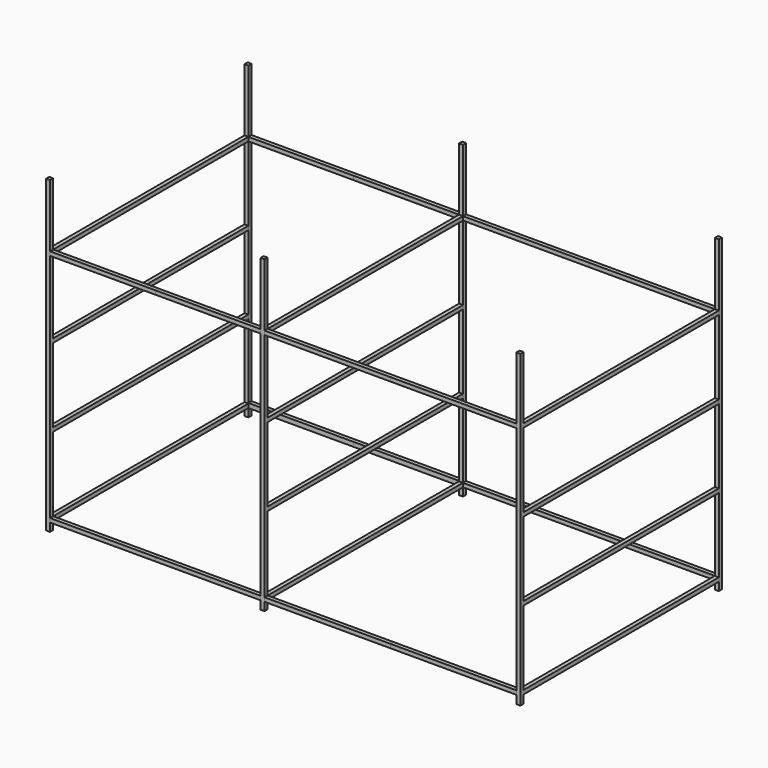
from build123d import *

# Parameters (mm, degrees)
F0_W      = 38.1
F0_H      = 3000
F1_DEPTH  = 38.1
F2_W      = 38.1
F2_H      = 38.1
F3_DEPTH  = 2363.8
F4_W      = 38.1
F4_H      = 38.1
F5_DEPTH  = 2363.8
F6_W      = 38.1
F6_H      = 38.1
F7_DEPTH  = 2363.8
F8_W      = 38.1
F8_H      = 38.1
F9_DEPTH  = 1020
F8_H_2    = 42.8596847504
F11_W     = 38.1
F11_H     = 38.1
F12_DEPTH = 1220


with BuildPart() as f1:
    # F0 (on Right) → F1 (new body)
    with BuildSketch(Plane.YZ):
        with Locations((-185.9003488964, 11.6033870727)):
            Rectangle(F0_W, F0_H)
    extrude(amount=F1_DEPTH)

    # F2 (on face) → F3 (join)
    with BuildSketch(Plane(origin=(0, -166.8503488964, 0), x_dir=(-1, 0, 0), z_dir=(0, 1, 0))):
        with Locations((-19.05, -1389.3466129273)):
            Rectangle(F2_W, F2_H)
    extrude(amount=F3_DEPTH)

    # F4 (on face) → F5 (join)
    with BuildSketch(Plane(origin=(0, -166.8503488964, 0), x_dir=(-1, 0, 0), z_dir=(0, 1, 0))):
        with Locations((-19.05, -631.2466129273)):
            Rectangle(F4_W, F4_H)
    extrude(amount=F5_DEPTH)

    # F6 (on face) → F7 (join)
    with BuildSketch(Plane(origin=(0, -166.8503488964, 0), x_dir=(-1, 0, 0), z_dir=(0, 1, 0))):
        with Locations((-19.05, 126.8533870727)):
            Rectangle(F6_W, F6_H)
        with Locations((-19.05, 884.9533870727)):
            Rectangle(F6_W, F6_H)
    extrude(amount=F7_DEPTH)


with BuildPart() as f1b:
    # F0 (on Right) → F1, piece 2 (new body)
    with BuildSketch(Plane.YZ):
        with Locations((2215.9996511036, 11.6033870727)):
            Rectangle(F0_W, F0_H)
    extrude(amount=F1_DEPTH)


with BuildPart() as f9:
    # F8 (on face) → F9 (new body)
    with BuildSketch(Plane(origin=(0, 0, 0), x_dir=(0, -1, 0), z_dir=(-1, 0, 0))):
        with Locations((185.9003488964, 884.9533870727)):
            Rectangle(F8_W, F8_H)
    extrude(amount=F9_DEPTH)


with BuildPart() as f9b:
    # F8 (on face) → F9, piece 2 (new body)
    with BuildSketch(Plane(origin=(0, 0, 0), x_dir=(0, -1, 0), z_dir=(-1, 0, 0))):
        with Locations((-2215.9996511036, 884.9533870727)):
            Rectangle(F8_W, F8_H)
    extrude(amount=F9_DEPTH)


with BuildPart() as f9c:
    # F8 (on face) → F9, piece 3 (new body)
    with BuildSketch(Plane(origin=(0, 0, 0), x_dir=(0, -1, 0), z_dir=(-1, 0, 0))):
        with Locations((-2215.9996511036, -1386.9667705521)):
            Rectangle(F8_W, F8_H_2)
    extrude(amount=F9_DEPTH)


with BuildPart() as f9d:
    # F8 (on face) → F9, piece 4 (new body)
    with BuildSketch(Plane(origin=(0, 0, 0), x_dir=(0, -1, 0), z_dir=(-1, 0, 0))):
        with Locations((185.9003488964, -1389.3466129273)):
            Rectangle(F8_W, F8_H)
    extrude(amount=F9_DEPTH)


with BuildPart() as f10_1:
    # F10: instance of F1
    add(f1.part.mirror(Plane(origin=(-1020, 2215.9996511036, 884.9533870727), x_dir=(0, -1, 0), z_dir=(-1, 0, 0))))


with BuildPart() as f10_2:
    # F10: instance of F1b
    add(f1b.part.mirror(Plane(origin=(-1020, 2215.9996511036, 884.9533870727), x_dir=(0, -1, 0), z_dir=(-1, 0, 0))))


with BuildPart() as f10_3:
    # F10: instance of F9
    add(f9.part.mirror(Plane(origin=(-1020, 2215.9996511036, 884.9533870727), x_dir=(0, -1, 0), z_dir=(-1, 0, 0))))


with BuildPart() as f10_4:
    # F10: instance of F9b
    add(f9b.part.mirror(Plane(origin=(-1020, 2215.9996511036, 884.9533870727), x_dir=(0, -1, 0), z_dir=(-1, 0, 0))))


with BuildPart() as f10_5:
    # F10: instance of F9c
    add(f9c.part.mirror(Plane(origin=(-1020, 2215.9996511036, 884.9533870727), x_dir=(0, -1, 0), z_dir=(-1, 0, 0))))


with BuildPart() as f10_6:
    # F10: instance of F9d
    add(f9d.part.mirror(Plane(origin=(-1020, 2215.9996511036, 884.9533870727), x_dir=(0, -1, 0), z_dir=(-1, 0, 0))))


with BuildPart() as f12:
    # F11 (on face) → F12 (new body)
    with BuildSketch(Plane.YZ.offset(38.1)):
        with Locations((-185.9003488964, 884.9533870727)):
            Rectangle(F11_W, F11_H)
    extrude(amount=F12_DEPTH)


with BuildPart() as f12b:
    # F11 (on face) → F12, piece 2 (new body)
    with BuildSketch(Plane.YZ.offset(38.1)):
        with Locations((2215.9996511036, 884.9533870727)):
            Rectangle(F11_W, F11_H)
    extrude(amount=F12_DEPTH)


with BuildPart() as f12c:
    # F11 (on face) → F12, piece 3 (new body)
    with BuildSketch(Plane.YZ.offset(38.1)):
        with Locations((-185.9003488964, -1389.3466129273)):
            Rectangle(F11_W, F11_H)
    extrude(amount=F12_DEPTH)


with BuildPart() as f12d:
    # F11 (on face) → F12, piece 4 (new body)
    with BuildSketch(Plane.YZ.offset(38.1)):
        with Locations((2215.9996511036, -1389.3466129273)):
            Rectangle(F11_W, F11_H)
    extrude(amount=F12_DEPTH)


with BuildPart() as f13_1:
    # F13: instance of F1
    add(f1.part.mirror(Plane(origin=(1258.1, -185.9003488964, 884.9533870727), x_dir=(0, 1, 0), z_dir=(1, 0, 0))))


with BuildPart() as f13_2:
    # F13: instance of F1b
    add(f1b.part.mirror(Plane(origin=(1258.1, -185.9003488964, 884.9533870727), x_dir=(0, 1, 0), z_dir=(1, 0, 0))))


with BuildPart() as f13_3:
    # F13: instance of F12d
    add(f12d.part.mirror(Plane(origin=(1258.1, -185.9003488964, 884.9533870727), x_dir=(0, 1, 0), z_dir=(1, 0, 0))))


with BuildPart() as f13_4:
    # F13: instance of F12c
    add(f12c.part.mirror(Plane(origin=(1258.1, -185.9003488964, 884.9533870727), x_dir=(0, 1, 0), z_dir=(1, 0, 0))))


with BuildPart() as f13_5:
    # F13: instance of F12b
    add(f12b.part.mirror(Plane(origin=(1258.1, -185.9003488964, 884.9533870727), x_dir=(0, 1, 0), z_dir=(1, 0, 0))))


with BuildPart() as f13_6:
    # F13: instance of F12
    add(f12.part.mirror(Plane(origin=(1258.1, -185.9003488964, 884.9533870727), x_dir=(0, 1, 0), z_dir=(1, 0, 0))))


solid = Compound([f1.part, f1b.part, f9.part, f9b.part, f9c.part, f9d.part, f10_1.part, f10_2.part, f10_3.part, f10_4.part, f10_5.part, f10_6.part, f12.part, f12b.part, f12c.part, f12d.part, f13_1.part, f13_2.part, f13_3.part, f13_4.part, f13_5.part, f13_6.part])
